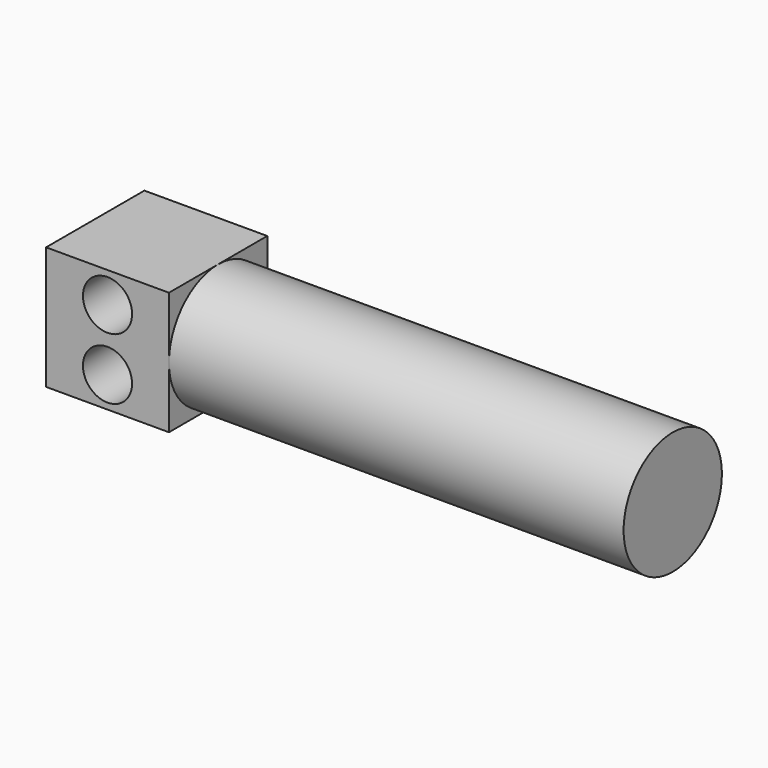
from build123d import *

# Parameters (mm, degrees)
F0_R     = 6.35
F1_DEPTH = 46.99328
F3_DEPTH = 12.7
F5_D     = 5.08
F5_DEPTH = 25.4
F5_TIP   = 1.5261859723


with BuildPart() as f1:
    # F0 (on Right) → F1 (new body)
    with BuildSketch(Plane.YZ):
        with Locations((42.2567352653, 52.6904910803)):
            Circle(F0_R)
    extrude(amount=F1_DEPTH)

    # F2 (on face) → F3 (join)
    with BuildSketch(Plane(origin=(0, 0, 0), x_dir=(0, -1, 0), z_dir=(-1, 0, 0))):
        with BuildLine():
            Line((-42.2567352653, 59.0404910803), (-48.6067352653, 59.0404910803))
            Line((-48.6067352653, 59.0404910803), (-48.6067352653, 52.6904910803))
            ThreePointArc((-48.6067352653, 52.6904910803), (-46.7468633258, 57.1806191408), (-42.2567352653, 59.0404910803))
        make_face()
        with BuildLine():
            Line((-35.9067352653, 59.0404910803), (-42.2567352653, 59.0404910803))
            ThreePointArc((-42.2567352653, 59.0404910803), (-37.7666072047, 57.1806191408), (-35.9067352653, 52.6904910803))
            Line((-35.9067352653, 52.6904910803), (-35.9067352653, 59.0404910803))
        make_face()
        with BuildLine():
            ThreePointArc((-35.9067352653, 52.6904910803), (-37.7666072047, 57.1806191408), (-42.2567352653, 59.0404910803))
            ThreePointArc((-42.2567352653, 59.0404910803), (-46.7468633258, 57.1806191408), (-48.6067352653, 52.6904910803))
            ThreePointArc((-48.6067352653, 52.6904910803), (-46.7468633258, 48.2003630197), (-42.2567352653, 46.3404910803))
            ThreePointArc((-42.2567352653, 46.3404910803), (-37.7666072047, 48.2003630197), (-35.9067352653, 52.6904910803))
        make_face()
        with BuildLine():
            ThreePointArc((-42.2567352653, 46.3404910803), (-46.7468633258, 48.2003630197), (-48.6067352653, 52.6904910803))
            Line((-48.6067352653, 52.6904910803), (-48.6067352653, 46.3404910803))
            Line((-48.6067352653, 46.3404910803), (-42.2567352653, 46.3404910803))
        make_face()
        with BuildLine():
            Line((-35.9067352653, 46.3404910803), (-35.9067352653, 52.6904910803))
            ThreePointArc((-35.9067352653, 52.6904910803), (-37.7666072047, 48.2003630197), (-42.2567352653, 46.3404910803))
            Line((-42.2567352653, 46.3404910803), (-35.9067352653, 46.3404910803))
        make_face()
    extrude(amount=F3_DEPTH)

    # F5
    with Locations(Plane(origin=(0, 48.6067352653, 0), x_dir=(-1, 0, 0), z_dir=(0, 1, 0))):
        with Locations((6.35, 55.8654910803), (6.35, 49.5154910803)):
            Hole(F5_D / 2, depth=F5_DEPTH)
            with Locations((0, 0, -(F5_DEPTH + F5_TIP / 2))):  # 118° drill point
                Cone(0, F5_D / 2, F5_TIP, mode=Mode.SUBTRACT)


solid = f1.part
